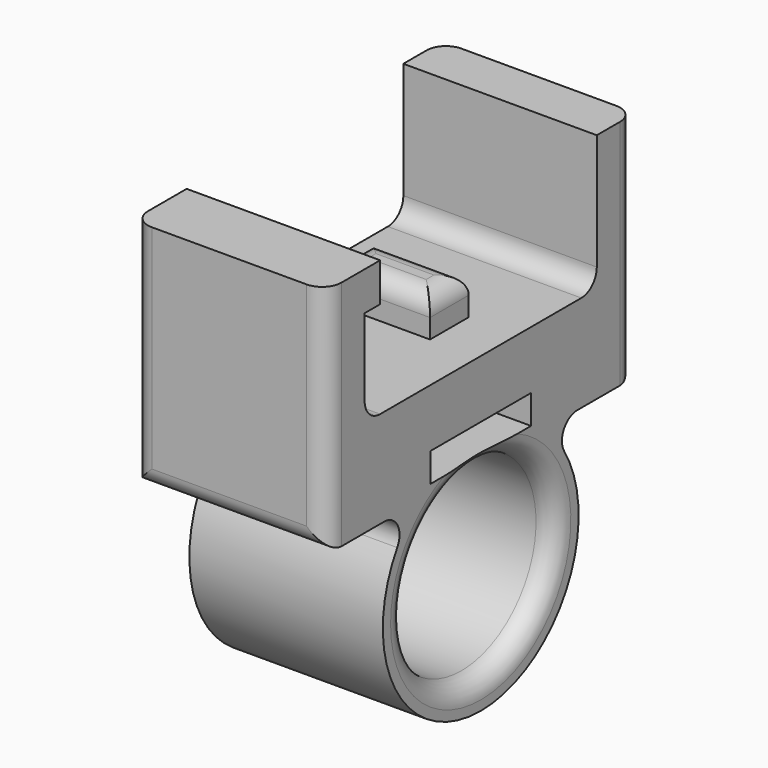
from build123d import *

# Parameters (mm, degrees)
F0_W         = 10
F0_H         = 20
F1_DEPTH     = 5
F2_W         = 10
F2_H         = 2.5
F3_DEPTH     = 7
F4_W         = 10
F4_H         = 2
F5_DEPTH     = 1
F6_W         = 5
F6_H         = 2.5
F7_DEPTH     = 2
F8_R         = 1
F9_W         = 6.5
F9_H         = 1.5
F10_DEPTH    = 10.001
F12_DEPTH    = 5
F13_R        = 4.825
F14_DEPTH    = 10.001
F15_T1_DEPTH = 10


# Not quite as in the source:
# - a fillet or chamfer that OpenCascade refuses, or shapes differently, is made with other operations: its cross-section is extruded or revolved along the edge and cut away or added


with BuildPart() as f1:
    # F0 (on Top) → F1 (new body)
    with BuildSketch(Plane.XY):
        Rectangle(F0_W, F0_H)
    extrude(amount=F1_DEPTH)

    # F2 (on face) → F3 (join)
    with BuildSketch(Plane.XY.offset(5)):
        with Locations((0, -8.75)):
            Rectangle(F2_W, F2_H)
        with Locations((0, 8.75)):
            Rectangle(F2_W, F2_H)
    extrude(amount=F3_DEPTH)

    # F4 (on face) → F5 (join)
    with BuildSketch(Plane(origin=(0, -7.5, 0), x_dir=(-1, 0, 0), z_dir=(0, 1, 0))):
        with Locations((0, 11)):
            Rectangle(F4_W, F4_H)
    extrude(amount=F5_DEPTH)

    # F6 (on face) → F7 (join)
    with BuildSketch(Plane.XY.offset(5)):
        with Locations((0, 1.1)):
            Rectangle(F6_W, F6_H)
    extrude(amount=F7_DEPTH)

    # F8
    f8_edges = [f1.edges().sort_by_distance(p)[0] for p in [
        (0, 7.5, 5),
        (0, -7.5, 5),
        (0, 10, 0),
        (0, -10, 0),
        (5, -10, 6),
        (-5, -10, 6),
        (5, 10, 6),
        (-5, 10, 6),
        (2.5, 1.1, 7),
        (0, 2.35, 7),
        (-2.5, 1.1, 7),
        (0, -0.15, 7),
    ]]
    fillet(f8_edges, radius=F8_R)

    # F9 (on face) → F10 (cut, through all)
    with BuildSketch(Plane.YZ.offset(5)):
        with Locations((0, 1.25)):
            Rectangle(F9_W, F9_H)
    extrude(amount=-F10_DEPTH, mode=Mode.SUBTRACT)

    # F11 (on Right) → F12 (join, symmetric)
    with BuildSketch(Plane.YZ):
        with BuildLine():
            Line((4.0896210093, 0), (0, 0))
            Line((0, 0), (-4.0896210093, 0))
            ThreePointArc((-4.0896210093, 0), (0, -11.15), (4.0896210093, 0))
        make_face()
        with BuildLine():
            ThreePointArc((0, 0), (3.4117902192, -1.4132097808), (4.825, -4.825))
            ThreePointArc((4.825, -4.825), (-3.4117902192, -8.2367902192), (0, 0))
        make_face(mode=Mode.SUBTRACT)
        with BuildLine():
            ThreePointArc((0, 0), (-3.4117902192, -8.2367902192), (4.825, -4.825))
            ThreePointArc((4.825, -4.825), (3.4117902192, -1.4132097808), (0, 0))
        make_face()
    extrude(amount=F12_DEPTH, both=True)

    # F13 (on face) → F14 (cut, through all)
    with BuildSketch(Plane(origin=(-5, 0, 0), x_dir=(0, -1, 0), z_dir=(-1, 0, 0))):
        with Locations((0, -4.825)):
            Circle(F13_R)
    extrude(amount=-F14_DEPTH, mode=Mode.SUBTRACT)

    # F15: fillet of radius 1 on 4 edges, made by hand

    # F15_s2 → F15_t1 (join)
    with BuildSketch(Plane.YZ.offset(-5)):
        with BuildLine():
            ThreePointArc((-6.2469992797, 0), (-5.3745933247, -0.5112179935), (-5.3941666135, -1.5221843003))
            ThreePointArc((-5.3941666135, -1.5221843003), (-4.8025845312, -0.7090788613), (-4.0896210093, 0))
            Line((-4.0896210093, 0), (-6.2469992797, 0))
        make_face()
        with BuildLine():
            ThreePointArc((6.2469992797, 0), (5.3745933247, -0.5112179935), (5.3941666135, -1.5221843003))
            ThreePointArc((5.3941666135, -1.5221843003), (4.8025845312, -0.7090788613), (4.0896210093, 0))
            Line((4.0896210093, 0), (6.2469992797, 0))
        make_face()
    extrude(amount=F15_T1_DEPTH)

    # F15_s3 → F15_t4 (revolve, cut)
    with BuildSketch(Plane.XY.offset(-4.825)):
        with BuildLine():
            ThreePointArc((-5, -5.825), (-4.7071067812, -5.1178932188), (-4, -4.825))
            Line((-4, -4.825), (-5, -4.825))
            Line((-5, -4.825), (-5, -5.825))
        make_face()
    revolve(axis=Axis((-5, 0, -4.825), (-1, 0, 0)), mode=Mode.SUBTRACT)

    # F15_s5 → F15_t6 (revolve, cut)
    with BuildSketch(Plane.XY.offset(-4.825)):
        with BuildLine():
            ThreePointArc((5, -5.825), (4.7071067812, -5.1178932188), (4, -4.825))
            Line((4, -4.825), (5, -4.825))
            Line((5, -4.825), (5, -5.825))
        make_face()
    revolve(axis=Axis((5, 0, -4.825), (-1, 0, 0)), mode=Mode.SUBTRACT)


solid = f1.part
